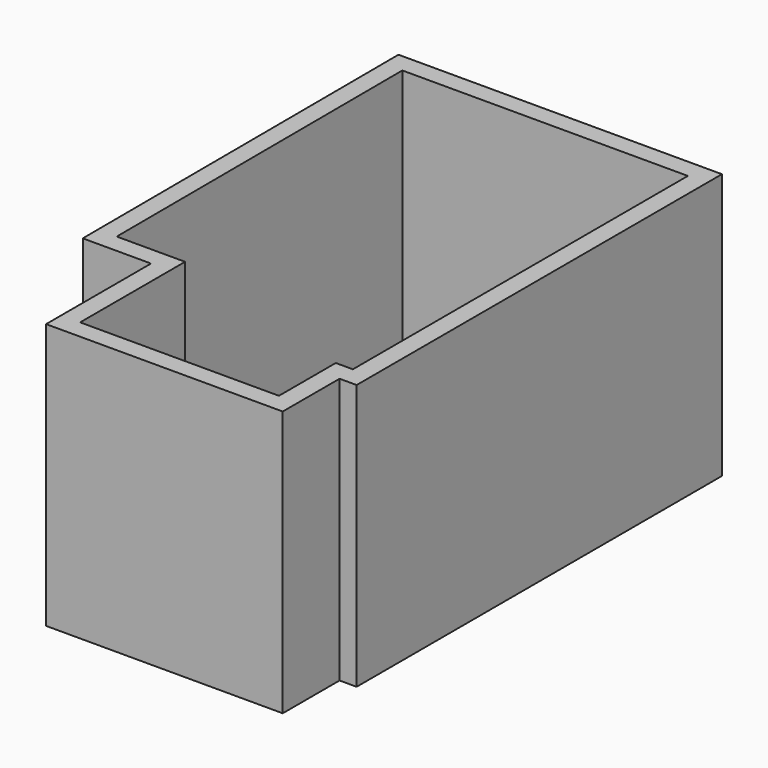
from build123d import *

# Parameters (mm, degrees)
F1_DEPTH = 2800
F2_W     = 900
F2_H     = 2000
F3_DEPTH = 199.3887424469


# Not quite as in the source:
# - a feature of the source that left no trace in its solid (it failed there, or was rolled back) is left out


with BuildPart() as f1:
    # F0 (on Top) → F1 (new body)
    with BuildSketch(Plane.XY):
        Polygon((1537.0936393738, -5293.5702800751), (1537.0936393738, -4544.8143482208), (1717.0830965042, -4544.8143482208), (1717.0830965042, 267.3035189509), (-1691.8783106137, 267.3035189509), (-1675.9599854953, -3911.2515449524), (-956.7605257034, -3911.2515449524), (-956.7605257034, -5293.5702800751), align=None)
        Polygon((-757.3717832565, -3711.8628025055), (-1477.3293733597, -3711.8628025055), (-1491.7285442352, 67.914776504), (1517.6943540573, 67.914776504), (1517.6943540573, -4345.4256057739), (1337.7048969269, -4345.4256057739), (1337.7048969269, -5094.1815376282), (-757.3717832565, -5094.1815376282), align=None, mode=Mode.SUBTRACT)
    extrude(amount=F1_DEPTH)

    # F2 (on face) → F3 (cut, through all)
    with BuildSketch(Plane(origin=(-956.7605257034, 0, 0), x_dir=(0, -1, 0), z_dir=(-1, 0, 0))):
        with Locations((4463.5073661804, 1000)):
            Rectangle(F2_W, F2_H)
    extrude(amount=-F3_DEPTH, mode=Mode.SUBTRACT)


solid = f1.part
